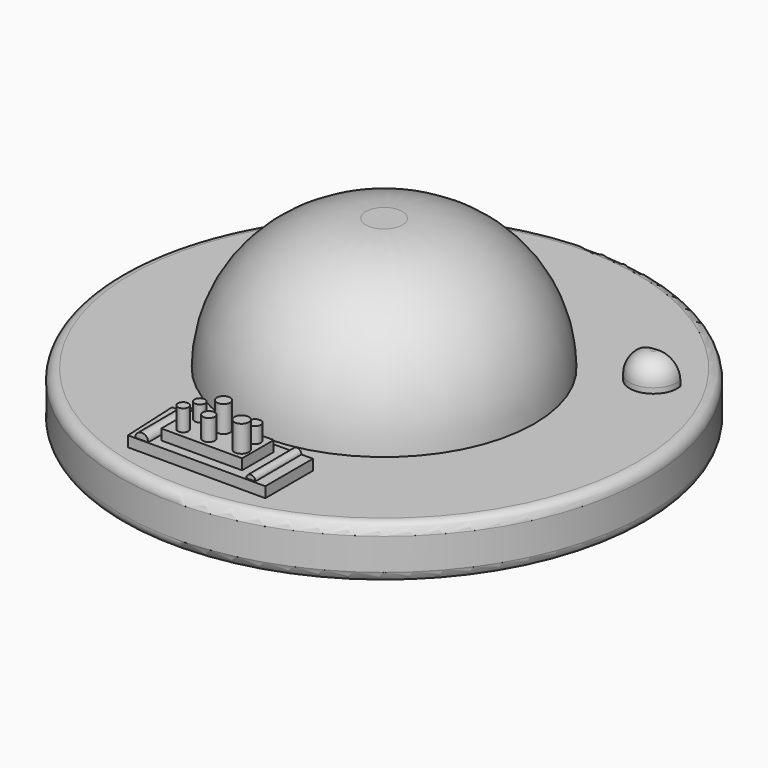
from build123d import *

# Parameters (mm, degrees)
F0_R      = 50
F1_DEPTH  = 10
F2_R      = 2
F3_R      = 28.456793416
F4_DEPTH  = 25
F5_R      = 24.99999
F6_R      = 4.5
F7_DEPTH  = 5
F9_DEPTH  = 5
F10_R     = 4
F12_DEPTH = 5
F13_R     = 4
F15_DEPTH = 2
F16_R     = 0.8595542321
F16_R_2   = 1.219346416
F17_DEPTH = 11
F18_W     = 15.3063726611
F18_H     = 7.4906051159
F19_DEPTH = 2
F20_R     = 1.3613365602
F20_R_2   = 1.2793093954
F21_DEPTH = 5
F20_R_3   = 1.0051427106
F20_R_4   = 1.1191673647
F22_DEPTH = 3
F20_R_5   = 1.0069734003
F20_R_6   = 1.1374722919
F23_DEPTH = 4


# Not quite as in the source:
# - a fillet or chamfer is up to 0.001 mm smaller than in the source, because OpenCascade refuses the exact size


with BuildPart() as f1:
    # F0 (on Top) → F1 (new body)
    with BuildSketch(Plane.XY):
        Circle(F0_R)
    extrude(amount=F1_DEPTH)

    # F2
    f2_edges = [f1.edges().sort_by_distance(p)[0] for p in [
        (-50, 0, 10),
        (-50, 0, 0),
    ]]
    fillet(f2_edges, radius=F2_R)

    # F3 (on face) → F4 (join)
    with BuildSketch(Plane.XY.offset(10)):
        Circle(F3_R)
    extrude(amount=F4_DEPTH)

    # F5 (radius 25 in the source; OpenCascade refuses exactly that, so slightly less here)
    f5_edges = [f1.edges().sort_by_distance(p)[0] for p in [
        (-28.456793, 0, 35),
    ]]
    fillet(f5_edges, radius=F5_R)

    # F6 (on face) → F7 (join)
    with BuildSketch(Plane.XY.offset(10)):
        with Locations((-31.595224242, 24.5304261092)):
            Circle(F6_R)
        with Locations((33.404775758, 22.0027488409)):
            Circle(F6_R)
    extrude(amount=F7_DEPTH)

    # F8 (on face) → F9 (cut)
    with BuildSketch(Plane.XY.offset(15)):
        with BuildLine():
            Line((28.9127137026, 21.7355813083), (37.8271397629, 22.8350328115))
            ThreePointArc((37.8271397629, 22.8350328115), (32.8360512403, 26.6140051327), (28.9127137026, 21.7355813083))
        make_face()
        with BuildLine():
            Line((28.9127137026, 21.7355813083), (37.8271397629, 22.8350328115))
            ThreePointArc((37.8271397629, 22.8350328115), (32.8539465135, 26.4689090646), (28.9127137026, 21.7355813083))
        make_face()
    extrude(amount=-F9_DEPTH, mode=Mode.SUBTRACT)

    # F10
    f10_edges = [f1.edges().sort_by_distance(p)[0] for p in [
        (33.955605, 17.536589, 15),
    ]]
    fillet(f10_edges, radius=F10_R)

    # F11 (on face) → F12 (cut)
    with BuildSketch(Plane.XY.offset(15)):
        with BuildLine():
            Line((-36.0353056642, 25.2623256677), (-27.0957896794, 24.6017606519))
            ThreePointArc((-27.0957896794, 24.6017606519), (-31.2565181281, 29.1141819041), (-36.0353056642, 25.2623256677))
        make_face()
        with BuildLine():
            Line((-36.0353056642, 25.2623256677), (-27.0957896794, 24.6017606519))
            ThreePointArc((-27.0957896794, 24.6017606519), (-31.2636111635, 29.0181908942), (-36.0353056642, 25.2623256677))
        make_face()
    extrude(amount=-F12_DEPTH, mode=Mode.SUBTRACT)

    # F13
    f13_edges = [f1.edges().sort_by_distance(p)[0] for p in [
        (-31.926837, 20.042661, 15),
    ]]
    fillet(f13_edges, radius=F13_R)

    # F14 (on face) → F15 (join)
    with BuildSketch(Plane.XY.offset(10)):
        Polygon((-13.7490294874, -43.4411987662), (12.2883236036, -43.4879809618), (12.2883236036, -32.2040617466), (-14.2757371068, -32.3610827327), align=None)
    extrude(amount=F15_DEPTH)

    # F16 (on face) → F17 (join)
    with BuildSketch(Plane(origin=(0.1907818986, -32.2755706905, 0), x_dir=(-0.9999825303, -0.0059109277, 0), z_dir=(-0.0059109277, 0.9999825303, 0))):
        with Locations((-9.0753892437, 12)):
            Circle(F16_R)
        with Locations((11.4709548652, 12)):
            Circle(F16_R_2)
    extrude(amount=-F17_DEPTH)

    # F18 (on face) → F19 (join)
    with BuildSketch(Plane.XY.offset(12)):
        with Locations((-1.2223811354, -37.9079021513)):
            Rectangle(F18_W, F18_H)
    extrude(amount=F19_DEPTH)

    # F20 (on face) → F21 (join)
    with BuildSketch(Plane.XY.offset(14)):
        with Locations((4.6129520051, -39.5028851926)):
            Circle(F20_R)
        with Locations((-1.3699786505, -36.3012962043)):
            Circle(F20_R_2)
    extrude(amount=F21_DEPTH)

    # F20 (on face) → F22 (join)
    with BuildSketch(Plane.XY.offset(14)):
        with Locations((-6.2384037301, -35.8086153865)):
            Circle(F20_R_3)
        with Locations((4.3789707124, -36.0359735787)):
            Circle(F20_R_4)
    extrude(amount=F22_DEPTH)

    # F20 (on face) → F23 (join)
    with BuildSketch(Plane.XY.offset(14)):
        with Locations((-6.1916210689, -39.8297198117)):
            Circle(F20_R_5)
        with Locations((-1.3725927565, -39.7753641009)):
            Circle(F20_R_6)
    extrude(amount=F23_DEPTH)


solid = f1.part
